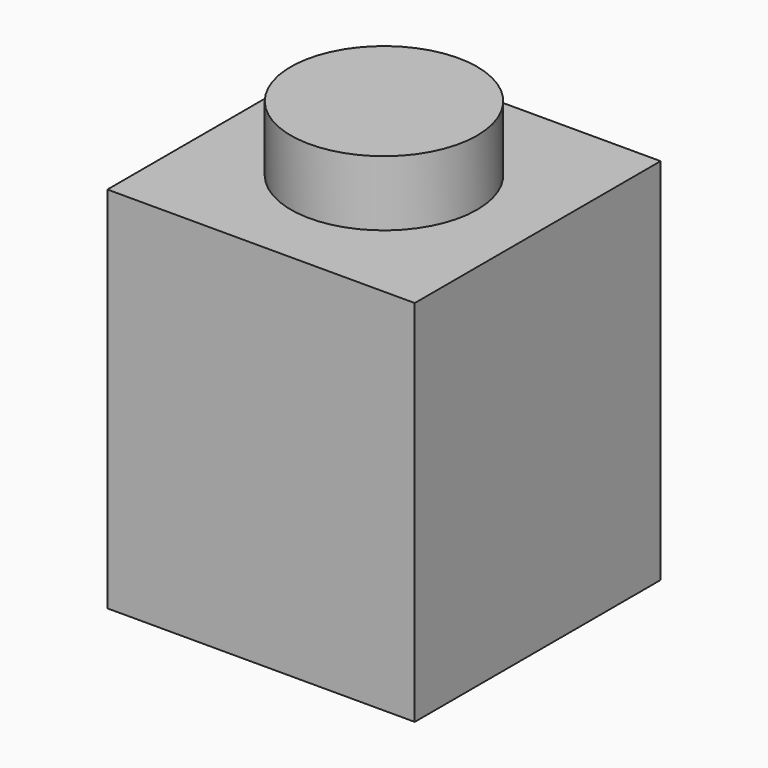
from build123d import *

# Parameters (mm, degrees)
F0_W     = 8.001
F0_H     = 8
F1_DEPTH = 9.6
F2_R     = 2.425
F3_DEPTH = 1.7
F4_T     = -1.5


with BuildPart() as f1:
    # F0 (on Top) → F1 (new body)
    with BuildSketch(Plane.XY):
        Rectangle(F0_W, F0_H)
    extrude(amount=F1_DEPTH)

    # F2 (on face) → F3 (join)
    with BuildSketch(Plane.XY.offset(9.6)):
        Circle(F2_R)
    extrude(amount=F3_DEPTH)

    # F4
    f4_openings = [f1.faces().sort_by_distance(p)[0] for p in [
        (0, 0, 0),
    ]]
    offset(amount=F4_T, openings=f4_openings, kind=Kind.INTERSECTION)


solid = f1.part
